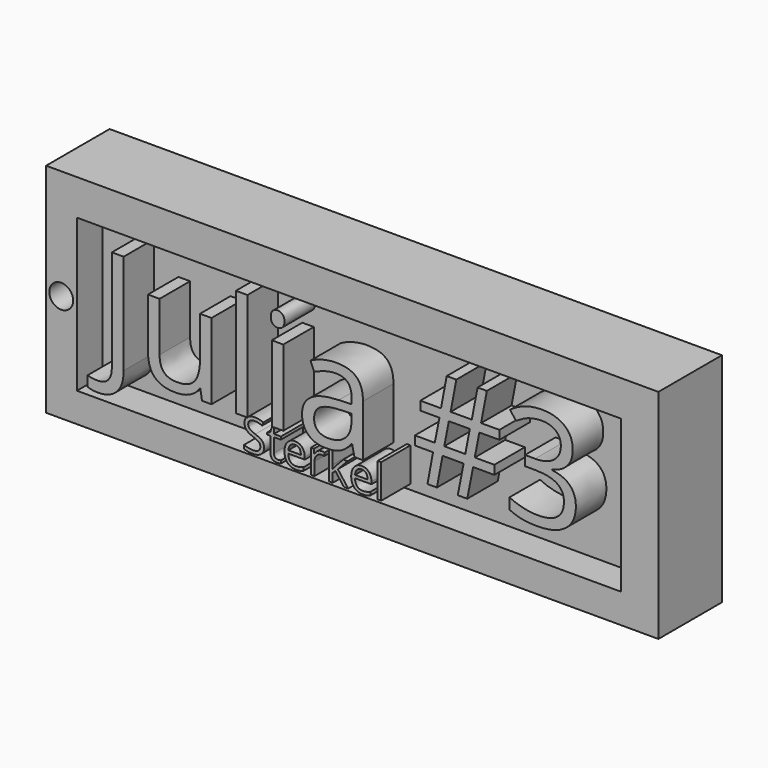
from build123d import *

# Parameters (mm, degrees)
F0_W         = 97.9557484388
F0_H         = 34.8000694066
F0_W_2       = 87.0037972927
F0_H_2       = 24.3743099272
F1_DEPTH     = 12.7
F2_W         = 87.2678272426
F2_H         = 25.0269109383
F3_DEPTH     = 7.62
F4_TEXT_SIZE = 22.7073129887
F5_DEPTH     = 13.716
F7_D         = 3.81
F8_TEXT_SIZE = 7.1422500898
F9_DEPTH     = 13.462


# Not quite as in the source:
# - Text() gives the source's letters only with a copy of the font that has no kerning and outlines rounded to 1/6400 em; it was checked with that copy


with BuildPart() as f1:
    # F0 (on Front) → F1 (new body)
    with BuildSketch(Plane.XZ):
        with Locations((-4.4086277485, 0.1962343231)):
            Rectangle(F0_W, F0_H)
        with Locations((-4.9474798143, -0.3033578396)):
            Rectangle(F0_W_2, F0_H_2, mode=Mode.SUBTRACT)
    extrude(amount=F1_DEPTH)

    # F2 (on Front) → F3 (join)
    with BuildSketch(Plane.XZ):
        with Locations((-5.023593083, -0.543944072)):
            Rectangle(F2_W, F2_H)
    extrude(amount=F3_DEPTH)

    # F4 (on Front) → F5 (join)
    with BuildSketch(Plane.XZ):
        with Locations((-44.1595427692, -6.7226202227)):
            Text('Julia #3', F4_TEXT_SIZE, font='Open Sans', text_align=(TextAlign.LEFT, TextAlign.BOTTOM))
    extrude(amount=F5_DEPTH)

    # F7 (through all)
    with Locations(Plane(origin=(0, 0, 0), x_dir=(1, 0, 0), z_dir=(0, 1, 0))):
        with Locations((-50.9630925953, 0)):
            Hole(F7_D / 2)

    # F8 (on Front) → F9 (join)
    with BuildSketch(Plane.XZ):
        with Locations((-21.4771647006, -11.646068655)):
            Text('Sterkel', F8_TEXT_SIZE, font='Open Sans', text_align=(TextAlign.LEFT, TextAlign.BOTTOM))
    extrude(amount=F9_DEPTH)


solid = f1.part
